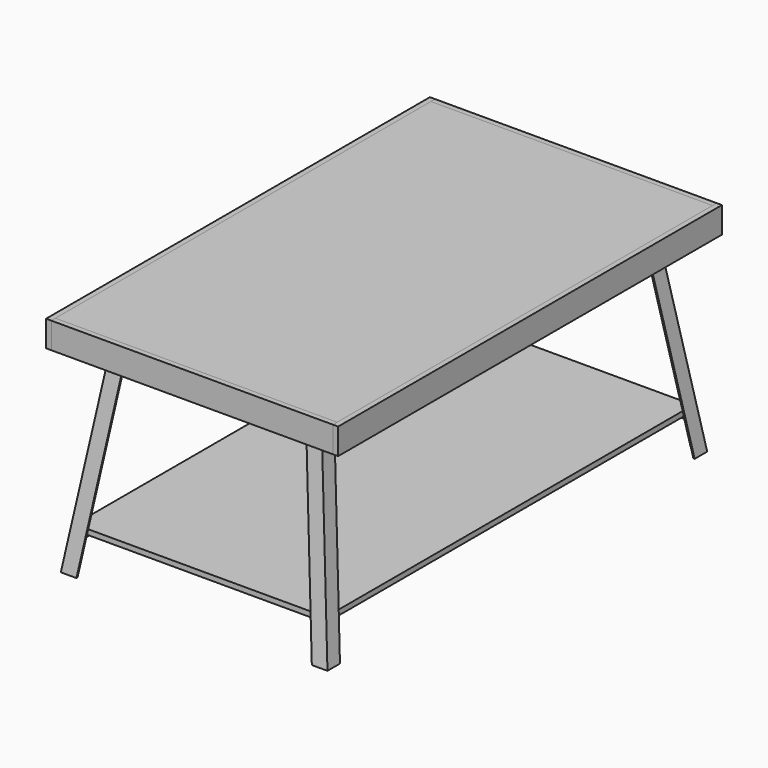
from build123d import *

# Parameters (mm, degrees)
F0_W      = 685.8
F0_H      = 1143
F1_DEPTH  = 25.4
F2_W      = 685.8
F2_H      = 12.7
F3_DEPTH  = 63.5
F4_DEPTH  = 63.5
F7_W      = 685.8
F7_H      = 63.5
F8_DEPTH  = 12.7
F13_W     = 609.6
F13_H     = 50.8
F14_DEPTH = 3.175
F18_DEPTH = 3.175
F21_W     = 34.925
F21_H     = 34.925
F22_DEPTH = 3.175
F25_W     = 611.4661372068
F25_H     = 1118.335616345
F26_DEPTH = 12.7


# Not quite as in the source:
# - a feature of the source that left no trace in its solid (it failed there, or was rolled back) is left out


with BuildPart() as f1:
    # F0 (on Top) → F1 (new body)
    with BuildSketch(Plane.XY):
        Rectangle(F0_W, F0_H)
    extrude(amount=F1_DEPTH)


with BuildPart() as f3:
    # F2 (on face) → F3 (new body)
    with BuildSketch(Plane.XY.offset(25.4)):
        with Locations((0, -577.85)):
            Rectangle(F2_W, F2_H)
    extrude(amount=-F3_DEPTH)


with BuildPart() as f4:
    # F2 (on face) → F4 (new body)
    with BuildSketch(Plane.XY.offset(25.4)):
        Polygon((-342.9, -584.2), (-342.9, -571.5), (-342.9, 571.5), (-342.9, 584.2), (-355.6, 584.2), (-355.6, -584.2), align=None)
    extrude(amount=-F4_DEPTH)


with BuildPart() as f5_1:
    # F5: instance of F4
    add(f4.part.mirror(Plane.YZ))


with BuildPart() as f6_1:
    # F6: instance of F3
    add(f3.part.mirror(Plane.XZ))


with BuildPart() as f8:
    # F7 (on face) → F8 (new body)
    with BuildSketch(Plane(origin=(0, 0, 0), x_dir=(1, 0, 0), z_dir=(0, 0, -1))):
        with Locations((0, 488.95)):
            Rectangle(F7_W, F7_H)
    extrude(amount=F8_DEPTH)


with BuildPart() as f8b:
    # F7 (on face) → F8, piece 2 (new body)
    with BuildSketch(Plane(origin=(0, 0, 0), x_dir=(1, 0, 0), z_dir=(0, 0, -1))):
        Rectangle(F7_W, F7_H)
    extrude(amount=F8_DEPTH)


with BuildPart() as f12:
    # F12: sweep along a path in F11
    with BuildLine(Plane(origin=(0, -496.4101735589, 69.7659001467), x_dir=(1, 0, 0), z_dir=(0, -0.9902680687, 0.139173101))) as f12_path:
        Line((-254, -83.2763397607), (-324.6999352877, -586.3325186814))
    # F9 (on face) → F12 (sweep)
    with BuildSketch(Plane(origin=(0, 0, -12.7), x_dir=(1, 0, 0), z_dir=(0, 0, -1))):
        Polygon((-254, 508), (-254, 469.9), (-250.825, 469.9), (-250.825, 504.825), (-215.9, 504.825), (-215.9, 508), align=None)
    sweep(path=f12_path.line)

    # F13 (on face) → F14 (join)
    with BuildSketch(Plane(origin=(0, 0, -12.7), x_dir=(1, 0, 0), z_dir=(0, 0, -1))):
        with Locations((0, 488.95)):
            Rectangle(F13_W, F13_H)
    extrude(amount=F14_DEPTH)

    # F16: F12 across plane


with BuildPart() as f12_1:
    add(f12.part)
    add(f12.part.mirror(Plane.YZ))


with BuildPart() as f18:
    # F17 (on face) → F18 (new body)
    with BuildSketch(Plane(origin=(0, -493.2966706166, 69.3283258444), x_dir=(-1, 0, 0), z_dir=(0, 0.9902680687, -0.139173101))):
        Polygon((297.1001110228, -412.0989890367), (-263.6480910569, -174.0754990191), (-267.1830878213, -199.2283079651), (301.0836328718, -440.4432197893), align=None)
    extrude(amount=F18_DEPTH)


with BuildPart() as f19_1:
    # F19: instance of F18
    add(f18.part.mirror(Plane.YZ))


with BuildPart() as f22:
    # F21 (on offset) → F22 (new body)
    with BuildSketch(Plane(origin=(0, 0, -421.9604707683), x_dir=(1, 0, 0), z_dir=(0, 0, -1))):
        with Locations((291.4455686034, 544.8803081725)):
            Rectangle(F21_W, F21_H)
    extrude(amount=F22_DEPTH)


with BuildPart() as f23_1:
    # F23: instance of F22
    add(f22.part.mirror(Plane.YZ))


with BuildPart() as f24_1:
    # F24: instance of F8
    add(f8.part.mirror(Plane.XZ))


with BuildPart() as f24_2:
    # F24: instance of F12
    add(f12_1.part.mirror(Plane.XZ))


with BuildPart() as f24_3:
    # F24: instance of F19_1
    add(f19_1.part.mirror(Plane.XZ))


with BuildPart() as f24_4:
    # F24: instance of F18
    add(f18.part.mirror(Plane.XZ))


with BuildPart() as f24_5:
    # F24: instance of F23_1
    add(f23_1.part.mirror(Plane.XZ))


with BuildPart() as f24_6:
    # F24: instance of F22
    add(f22.part.mirror(Plane.XZ))


with BuildPart() as f26:
    # F25 (on face) → F26 (new body)
    with BuildSketch(Plane.XY.offset(-421.9604707683)):
        Rectangle(F25_W, F25_H)
    extrude(amount=F26_DEPTH)


solid = Compound([f1.part, f3.part, f4.part, f5_1.part, f6_1.part, f8.part, f8b.part, f12_1.part, f22.part, f23_1.part, f24_1.part, f24_2.part, f24_5.part, f24_6.part, f26.part])
